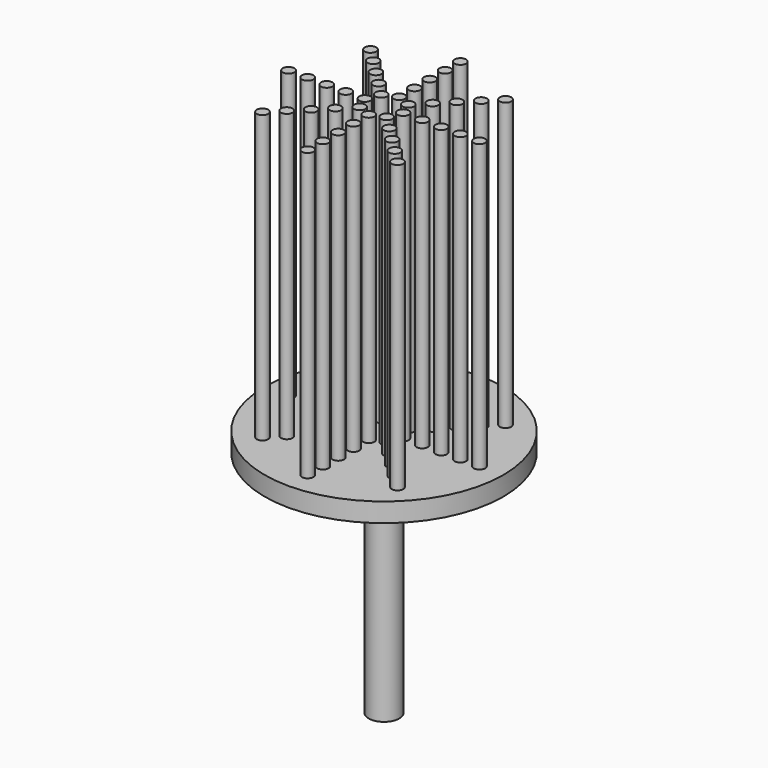
from build123d import *

# Parameters (mm, degrees)
F0_R            = 62.5
F1_DEPTH        = 10
F2_R            = 3
F3_DEPTH        = 150
F3_COPIES_COUNT = 8
F4_R            = 8
F5_DEPTH        = 120


# Not quite as in the source:
# - a pattern or mirror of a feature is missing from the dataset's text; its kind, count and spacing are read off the source's solid


with BuildPart() as f1:
    # F0 (on Top) → F1 (new body)
    with BuildSketch(Plane.XY):
        Circle(F0_R)
    extrude(amount=F1_DEPTH)

    # F2 (on face) → F3 (join)
    with BuildSketch(Plane.XY.offset(10)):
        with Locations((10, 0)):
            Circle(F2_R)
        with Locations((20, 0)):
            Circle(F2_R)
        with Locations((30, 0)):
            Circle(F2_R)
        with Locations((40, 0)):
            Circle(F2_R)
        with Locations((50, 0)):
            Circle(F2_R)
    f3 = extrude(amount=F3_DEPTH)

    # F3_copies: F3 ×8 about axis
    f3_copies_axis = Axis((0, 0, 0), (0, 0, 1))
    for i in range(1, F3_COPIES_COUNT):
        add(f3.rotate(f3_copies_axis, i * 360 / F3_COPIES_COUNT))

    # F4 (on face) → F5 (join)
    with BuildSketch(Plane.XY):
        Circle(F4_R)
    extrude(amount=-F5_DEPTH)


solid = f1.part
